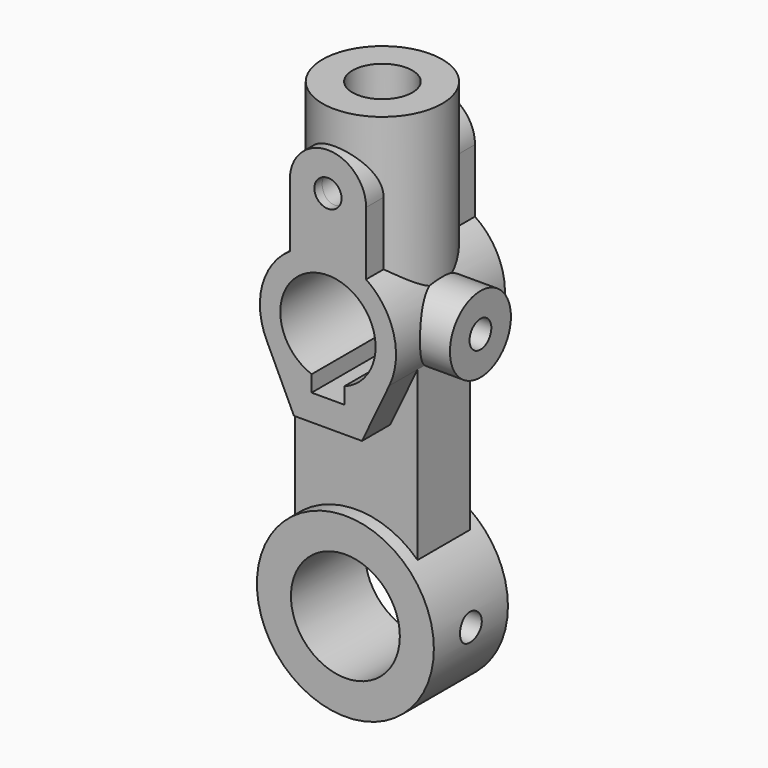
from build123d import *

# Parameters (mm, degrees)
F0_R           = 32.5
F0_R_2         = 20
F1_DEPTH       = 17
F2_R           = 5
F3_DEPTH       = 32.501
F5_DEPTH       = 12
F6_R           = 5
F7_DEPTH       = 25
F8_DEPTH       = 37.001
F10_R          = 22
F10_R_2        = 11
F11_DEPTH      = 70
F12_R          = 17.5
F12_R_2        = 5
F13_DEPTH      = 50.0010001
F16_END_RADIUS = 22
F15_R          = 14
F15_R_2        = 5
F16_REACH      = 108.0989798464


with BuildPart() as f1:
    # F0 (on Front) → F1 (new body, symmetric)
    with BuildSketch(Plane.XZ):
        Circle(F0_R)
        Circle(F0_R_2, mode=Mode.SUBTRACT)
    extrude(amount=F1_DEPTH, both=True)

    # F2 (on Right) → F3 (cut, through all)
    with BuildSketch(Plane.YZ):
        Circle(F2_R)
    extrude(amount=F3_DEPTH, mode=Mode.SUBTRACT)

    # F4 (on Front) → F5 (join, symmetric)
    with BuildSketch(Plane.XZ):
        with BuildLine():
            Line((-22.5, 96), (-22.5, 23.4520787991))
            ThreePointArc((-22.5, 23.4520787991), (0, 32.5), (22.5, 23.4520787991))
            Line((22.5, 23.4520787991), (22.5, 96))
            Line((22.5, 96), (-22.5, 96))
        make_face()
    extrude(amount=F5_DEPTH, both=True)

    # F6 (on Front) → F7 (join, symmetric)
    with BuildSketch(Plane.XZ):
        with BuildLine():
            Line((-22.5, 85.1027526411), (-12.5, 64))
            Line((-12.5, 64), (12.5, 64))
            Line((12.5, 64), (22.5, 85.1027526411))
            ThreePointArc((22.5, 85.1027526411), (24.1423613371, 102.4920250361), (14, 116.7123151772))
            Line((14, 116.7123151772), (14, 140))
            ThreePointArc((14, 140), (0, 154), (-14, 140))
            Line((-14, 140), (-14, 116.7123151772))
            ThreePointArc((-14, 116.7123151772), (-24.1423613371, 102.4920250361), (-22.5, 85.1027526411))
        make_face()
        with BuildLine():
            ThreePointArc((-6, 79.5607177772), (0, 113.5), (6, 79.5607177772))
            Line((6, 79.5607177772), (6, 73.6))
            Line((6, 73.6), (-6, 73.6))
            Line((-6, 73.6), (-6, 79.5607177772))
        make_face(mode=Mode.SUBTRACT)
        with Locations((0, 140)):
            Circle(F6_R, mode=Mode.SUBTRACT)
    extrude(amount=F7_DEPTH, both=True)

    # F8 (cut, through all): a face of the model
    f8_faces = [f1.faces().sort_by_distance(p)[0] for p in [
        (0, -12, 87.144181228),
    ]]
    extrude(f8_faces, amount=-F8_DEPTH, mode=Mode.SUBTRACT)

    # F10 (on offset) → F11 (join)
    with BuildSketch(Plane.XY.offset(96)):
        Circle(F10_R)
        Circle(F10_R_2, mode=Mode.SUBTRACT)
    extrude(amount=F11_DEPTH)

    # F12 (on face) → F13 (cut, through all)
    with BuildSketch(Plane.XZ.offset(25)):
        with Locations((0, 96)):
            Circle(F12_R)
        with Locations((0, 140)):
            Circle(F12_R_2)
    extrude(amount=-F13_DEPTH, mode=Mode.SUBTRACT)

    f16_end = (Plane(origin=(0, 0, 136.9371710435), x_dir=(-1, 0, 0), z_dir=(0, 0, -1)) * Cylinder(F16_END_RADIUS, 645.7430685017, mode=Mode.PRIVATE)).faces().sort_by_distance((-22, 0, 136.9371710435))[0]
    # F15 (on offset) → F16 (join, up to the whole of a round face its end follows)
    with BuildSketch(Plane.YZ.offset(36)):
        with Locations((0, 96)):
            Circle(F15_R)
        with Locations((0, 96)):
            Circle(F15_R_2, mode=Mode.SUBTRACT)
    f16_long = extrude(amount=-F16_REACH, mode=Mode.PRIVATE)
    add(split(f16_long, bisect_by=f16_end, keep=Keep.ALL, mode=Mode.PRIVATE).solids().sort_by_distance((36, -13.6040202025, 96))[0])


solid = f1.part
